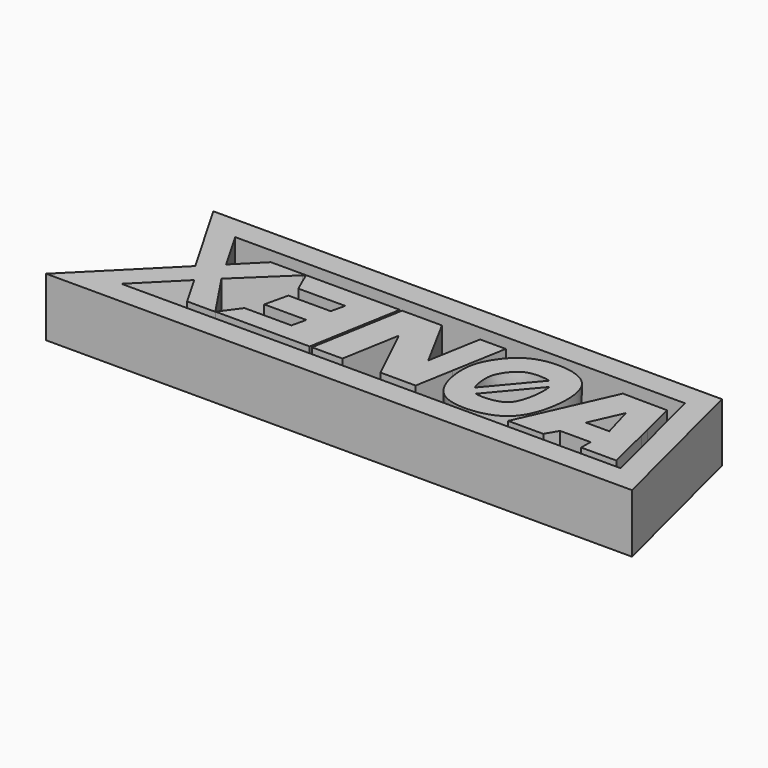
from build123d import *

# Parameters (mm, degrees)
F1_DEPTH = 25
F0_W     = 3.4720152617
F0_H     = 3.9200305776
F2_DEPTH = 15


# Not quite as in the source:
# - ends of sketch curves that miss each other by under 0.0002 mm in the source are joined
# - the dataset's text gives a spline's control points without its knots; the knots are read off the source's solid
# - a feature names something its author has since deleted; it is built from what else it names


with BuildPart() as f1:
    # F0 (on Top) → F1 (new body)
    with BuildSketch(Plane.XY):
        Polygon((35.3553390593, 35.3553390593), (0, 0), (250, 0), (232.3553390593, 69.9963552107), (15.3553390593, 69.9963552107), align=None)
        Polygon((149.3519097567, 59.9963530121), (224.56330661, 59.9963530121), (230.3136809852, 37.1846226695), (231.3968486735, 32.8876973548), (237.166372237, 10.0000021986), (140.1480585337, 10.0000021986), (136.676043272, 10.0000021986), (24.1421409317, 10.0000021986), (41.4001874912, 27.2580487582), (47.8522307846, 33.7100920516), (42.6758487445, 42.6758487445), (32.6758509431, 59.9963530121), (146.3302671909, 59.9963530121), align=None, mode=Mode.SUBTRACT)
        Polygon((53.2824504623, 53.2824504623), (42.6758487445, 42.6758487445), (47.8522307846, 33.7100920516), (67.4404504829, 52.4758059113), (68.2824504623, 53.2824504623), align=None)
        Polygon((60.8468717116, 14.278005959), (47.8522307846, 33.7100920516), (41.4001874912, 27.2580487582), (49.1933937334, 13.7598195929), (61.1933937334, 13.7598195929), align=None)
    extrude(amount=F1_DEPTH)


with BuildPart() as f1b:
    # F0 (on Top) → F1, piece 2 (new body)
    with BuildSketch(Plane.XY):
        Polygon((88.5540837341, 28.1308456181), (90.9036234209, 38.1308456181), (72.9036234209, 38.1308456181), (70.5540837341, 28.1308456181), align=None)
        Polygon((108.2824504623, 53.2824504623), (68.2824504623, 53.2824504623), (68.6377434378, 52.4758059113), (72.313347233, 44.1308456181), (92.313347233, 44.1308456181), (90.9036234209, 38.1308456181), (88.5540837341, 28.1308456181), (87.1034676285, 21.9568017674), (67.1034676285, 21.9568017674), (61.477565132, 14.278005959), (61.1933937334, 13.8901403418), (101.3365233556, 13.8901403418), align=None)
    extrude(amount=F1_DEPTH)



with BuildPart() as f1c:
    # F0 (on Top) → F1, piece 3 (new body)
    with BuildSketch(Plane.XY):
        Polygon((153.4814404268, 53.3123428967), (149.3519097567, 53.3123428967), (146.5191096067, 53.3123428967), (142.5191015005, 53.3123428967), (138.5251934142, 30.6617645774), (126.2824504623, 53.2824504623), (109.2824504623, 53.2824504623), (102.3365233556, 13.8901403418), (115.3365233556, 13.8901403418), (119.6777277973, 38.5103341671), (131.5355133201, 13.9200327762), (136.676043272, 13.9200327762), (140.1480585337, 13.9200327762), (146.5355133201, 13.9200327762), (149.3944048747, 30.1336124743), (151.5543764817, 42.3834201799), align=None)
    extrude(amount=F1_DEPTH)


with BuildPart() as f1d:
    # F0 (on Top) → F1, piece 4 (new body)
    with BuildSketch(Plane.XY):
        with BuildLine():
            add(Edge.make_bspline(
                [(153.2957728652, 41.0807725054), (153.49766281, 41.5309282211), (155.3500865512, 45.3378659555), (161.5552143615, 53.4867465492), (176.1548241084, 56.3217499328), (193.5548048204, 51.0510310034), (192.6995287251, 33.1029715051), (190.5478645245, 26.016644206)],
                knots=[0.0743708641, 0.0743708641, 0.0743708641, 0.0743708641, 0.0883183193, 0.1917010674, 0.3023367007, 0.4162516271, 0.5490950731, 0.5490950731, 0.5490950731, 0.5490950731], degree=3))
            add(Edge.make_bspline(
                [(151.5315026045, 33.6161878365), (151.6634499925, 36.3480245715), (152.2192517782, 38.6804443414), (153.2957728652, 41.0807725054)],
                knots=[0, 0, 0, 0, 0.0743708641, 0.0743708641, 0.0743708641, 0.0743708641], degree=3))
            add(Edge.make_bspline(
                [(151.5581660211, 30.4933039686), (151.4916370849, 31.5702465606), (151.4833764702, 32.6197850769), (151.5315026045, 33.6161878365)],
                knots=[0.9728741717, 0.9728741717, 0.9728741717, 0.9728741717, 1, 1, 1, 1], degree=3))
            add(Edge.make_bspline(
                [(188.4193204432, 20.8541177869), (186.4225620314, 17.2582664486), (179.6863041093, 11.4034157724), (160.3055787763, 10.4275817806), (153.2214749313, 20.0421386094), (151.7433054324, 27.4963446143), (151.5581660211, 30.4933039686)],
                knots=[0.5854070027, 0.5854070027, 0.5854070027, 0.5854070027, 0.6722296295, 0.7975352428, 0.8973873208, 0.9728741717, 0.9728741717, 0.9728741717, 0.9728741717], degree=3))
            add(Edge.make_bspline(
                [(190.5478645245, 26.016644206), (190.3967980643, 25.5191193687), (189.7761974015, 23.6315541865), (189.0399275657, 21.9717346898), (188.4193204432, 20.8541177869)],
                knots=[0.5490950731, 0.5490950731, 0.5490950731, 0.5490950731, 0.5584218951, 0.5854070027, 0.5854070027, 0.5854070027, 0.5854070027], degree=3))
        make_face()
        with BuildLine():
            add(Edge.make_bspline(
                [(162.8184250503, 25.0692523461), (162.7388528349, 25.2709199434), (162.5250729743, 25.8491123795), (162.2111113791, 26.8772771924), (161.811446171, 28.5859325459), (161.5680124914, 30.3698864013), (161.490617043, 32.0313577817), (161.5032118997, 32.7877081125), (161.5198585813, 33.1337514359)],
                knots=[0.8971962129, 0.8971962129, 0.8971962129, 0.8971962129, 0.90625, 0.921875, 0.9375, 0.96875, 0.984375, 1, 1, 1, 1], degree=3))
            add(Edge.make_bspline(
                [(161.5198585813, 33.1337514359), (161.5365052629, 33.4797947593), (161.5904971328, 34.1076177221), (161.7198338174, 34.8971109654), (161.8983772283, 35.617959176), (162.1037900469, 36.2305480911), (162.3191108206, 36.7643620724), (162.5109148317, 37.1933987719), (162.7379267984, 37.6574642255), (163.0921353714, 38.326605495), (163.596210236, 39.1811127594), (164.287470415, 40.1970519056), (165.0414513207, 41.1551577869), (165.8327231283, 42.017135319), (166.4983498938, 42.6285934344), (167.0176778213, 43.0428000772), (167.3981141086, 43.3156806379), (167.7595288983, 43.5467960735), (168.1488651256, 43.766963423), (168.5654607343, 43.9738592368), (169.1603655772, 44.23185257), (169.9804869671, 44.5178805652), (171.0896341478, 44.7915612101), (172.3184150489, 44.9834054828), (173.6559028444, 45.0826399089), (174.7295299917, 45.0813201083), (175.4692709806, 45.0471315589), (175.9685909899, 45.0153875781), (176.5764482855, 44.960404607), (177.2752413398, 44.8700053931), (178.152789541, 44.7188709988), (178.7412145092, 44.5732668808), (179.0910574906, 44.4674492213), (179.0945257888, 44.4663980322)],
                knots=[0, 0, 0, 0, 0.015625, 0.03125, 0.046875, 0.0625, 0.0703125, 0.078125, 0.0859375, 0.09375, 0.109375, 0.125, 0.140625, 0.15625, 0.171875, 0.1796875, 0.1875, 0.1953125, 0.203125, 0.2109375, 0.21875, 0.234375, 0.25, 0.265625, 0.28125, 0.296875, 0.30078125, 0.3046875, 0.3125, 0.3203125, 0.328125, 0.34375, 0.3439066519, 0.3439066519, 0.3439066519, 0.3439066519], degree=3))
            add(Edge.make_bspline(
                [(179.0945257888, 44.4663980322), (179.4369974189, 44.3626000224), (180.0408289592, 44.137858269), (180.6603332198, 43.8043498556), (180.954614815, 43.5775919437), (181.1038370269, 43.4315691806), (181.1895827034, 43.3310307887), (181.2538264485, 43.2395291398), (181.3046724038, 43.1550069204), (181.3582155541, 43.05569095), (181.422796919, 42.9212624239), (181.5199173994, 42.6948431225), (181.7085595453, 42.1772024114), (181.8753089955, 41.5231873988), (181.9696544415, 41.0096622148), (181.9730783847, 40.9907957298)],
                knots=[0.3439066519, 0.3439066519, 0.3439066519, 0.3439066519, 0.359375, 0.375, 0.390625, 0.3984375, 0.40625, 0.4140625, 0.41796875, 0.421875, 0.42578125, 0.4296875, 0.4375, 0.453125, 0.4537178211, 0.4537178211, 0.4537178211, 0.4537178211], degree=3))
            add(Edge.make_bspline(
                [(181.9730783847, 40.9907957298), (182.0598994005, 40.512397778), (182.2045363428, 39.41183358), (182.2797979507, 37.4823107399), (182.193566141, 35.3678582229), (181.9493626032, 33.2017921364), (181.5644163989, 31.0887847577), (181.0667847965, 29.1323622869), (180.5011449009, 27.4494312491), (179.9317447836, 26.1476864655), (179.3824865747, 25.1785905134), (178.8685398921, 24.4779841747), (178.3709172748, 23.9520794031), (177.8264944089, 23.5060953751), (177.1374617731, 23.0738355235), (176.2112022482, 22.6358864412), (174.9558716393, 22.2007569681), (173.4559950281, 21.8323747048), (171.8198374216, 21.5722282716), (170.1442177268, 21.4412866926), (168.5280439261, 21.4466193999), (167.3160139795, 21.558065936), (166.4822451641, 21.6958640201), (166.0986472535, 21.7808626756), (165.9163137021, 21.8272428827), (165.8971010414, 21.8322026836)],
                knots=[0.4537178211, 0.4537178211, 0.4537178211, 0.4537178211, 0.46875, 0.484375, 0.5, 0.515625, 0.53125, 0.546875, 0.5625, 0.578125, 0.59375, 0.609375, 0.625, 0.640625, 0.65625, 0.671875, 0.6875, 0.703125, 0.71875, 0.734375, 0.75, 0.765625, 0.7734375, 0.78125, 0.7821827292, 0.7821827292, 0.7821827292, 0.7821827292], degree=3))
            add(Edge.make_bspline(
                [(165.8971010414, 21.8322026836), (165.7553892759, 21.868785963), (165.5531970067, 21.9272567748), (165.3254056153, 22.0041417656), (165.1739060305, 22.0612615773), (165.0494707627, 22.1134592968), (164.8977695401, 22.1837784003), (164.7376634219, 22.2699020236), (164.5740601511, 22.3743238889), (164.3757102389, 22.5229923761), (164.1329229874, 22.7478764528), (163.795317607, 23.1578632169), (163.4078371213, 23.7696356085), (163.0732924198, 24.4470716455), (162.8761783378, 24.9228825776), (162.8184250503, 25.0692523461)],
                knots=[0.7821827292, 0.7821827292, 0.7821827292, 0.7821827292, 0.7890625, 0.79296875, 0.796875, 0.80078125, 0.8046875, 0.8125, 0.8203125, 0.828125, 0.84375, 0.859375, 0.875, 0.890625, 0.8971962129, 0.8971962129, 0.8971962129, 0.8971962129], degree=3))
        make_face(mode=Mode.SUBTRACT)
        with BuildLine():
            add(Edge.make_bspline(
                [(179.0945257888, 44.4663980322), (179.4369974189, 44.3626000224), (180.0408289592, 44.137858269), (180.6603332198, 43.8043498556), (180.954614815, 43.5775919437), (181.1038370269, 43.4315691806), (181.1895827034, 43.3310307887), (181.2538264485, 43.2395291398), (181.3046724038, 43.1550069204), (181.3582155541, 43.05569095), (181.422796919, 42.9212624239), (181.5199173994, 42.6948431225), (181.7085595453, 42.1772024114), (181.8753089955, 41.5231873988), (181.9696544415, 41.0096622148), (181.9730783847, 40.9907957298)],
                knots=[0.3439066519, 0.3439066519, 0.3439066519, 0.3439066519, 0.359375, 0.375, 0.390625, 0.3984375, 0.40625, 0.4140625, 0.41796875, 0.421875, 0.42578125, 0.4296875, 0.4375, 0.453125, 0.4537178211, 0.4537178211, 0.4537178211, 0.4537178211], degree=3))
            Line((179.0945257888, 44.4663980322), (162.8183697977, 25.0692305451))
            add(Edge.make_bspline(
                [(165.8971010414, 21.8322026836), (165.7553892759, 21.868785963), (165.5531970067, 21.9272567748), (165.3254056153, 22.0041417656), (165.1739060305, 22.0612615773), (165.0494707627, 22.1134592968), (164.8977695401, 22.1837784003), (164.7376634219, 22.2699020236), (164.5740601511, 22.3743238889), (164.3757102389, 22.5229923761), (164.1329229874, 22.7478764528), (163.795317607, 23.1578632169), (163.4078371213, 23.7696356085), (163.0732924198, 24.4470716455), (162.8761783378, 24.9228825776), (162.8183697977, 25.0692305451)],
                knots=[0.7821827292, 0.7821827292, 0.7821827292, 0.7821827292, 0.7890625, 0.79296875, 0.796875, 0.80078125, 0.8046875, 0.8125, 0.8203125, 0.828125, 0.84375, 0.859375, 0.875, 0.890625, 0.8971962129, 0.8971962129, 0.8971962129, 0.8971962129], degree=3))
            Line((165.8971010414, 21.8322026836), (181.9730783847, 40.9907957298))
        make_face()
    extrude(amount=F1_DEPTH)


with BuildPart() as f1e:
    # F0 (on Top) → F1, piece 5 (new body)
    with BuildSketch(Plane.XY):
        Polygon((227.8092346476, 32.8876973548), (226.7642129222, 37.1846226695), (223.0829559751, 52.321232543), (204.0839364723, 52.5142556785), (192.2389093289, 26.016644206), (189.1953905746, 19.20821933), (186.5355133201, 13.258009744), (201.5355133201, 13.258009744), (204.5355133201, 18.4541621667), (217.5355133201, 18.4541621667), (217.5355133201, 13.4541621667), (232.5355133201, 13.4541621667), align=None)
        Polygon((213.6570562804, 42.148201446), (217.5355133201, 28.4541621667), (207.5355133201, 28.4541621667), align=None, mode=Mode.SUBTRACT)
    extrude(amount=F1_DEPTH)


with BuildPart() as f1b_1:
    add(f1b.part)

    add(f1c.part)  # F2 merges F1c

    add(f1d.part)  # F2 merges F1d

    add(f1e.part)  # F2 merges F1e
    # F0 (on Top) → F2 (join)
    with BuildSketch(Plane.XY):
        Polygon((149.3519097567, 53.3123428967), (149.3519097567, 59.9963530121), (146.3302671909, 59.9963530121), (146.5191096067, 53.3123428967), align=None)
        with Locations((138.4120509028, 11.9600174874)):
            Rectangle(F0_W, F0_H)
        with BuildLine():
            Line((153.2957728652, 41.0807725054), (151.5543764817, 42.3834201799))
            Line((151.5543764817, 42.3834201799), (149.3944048747, 30.1336124743))
            Line((149.3944048747, 30.1336124743), (151.5581660211, 30.4933039686))
            add(Edge.make_bspline(
                [(151.5581660211, 30.4933039686), (151.4916370849, 31.5702465606), (151.4833764702, 32.6197850769), (151.5315026045, 33.6161878365)],
                knots=[0.9728741717, 0.9728741717, 0.9728741717, 0.9728741717, 1, 1, 1, 1], degree=3))
            add(Edge.make_bspline(
                [(151.5315026045, 33.6161878365), (151.6634499925, 36.3480245715), (152.2192517782, 38.6804443414), (153.2957728652, 41.0807725054)],
                knots=[0, 0, 0, 0, 0.0743708641, 0.0743708641, 0.0743708641, 0.0743708641], degree=3))
        make_face()
        with BuildLine():
            Line((189.1953905746, 19.20821933), (192.2389093289, 26.016644206))
            Line((192.2389093289, 26.016644206), (190.5478645245, 26.016644206))
            add(Edge.make_bspline(
                [(190.5478645245, 26.016644206), (190.3967980643, 25.5191193687), (189.7761974015, 23.6315541865), (189.0399275657, 21.9717346898), (188.4193204432, 20.8541177869)],
                knots=[0.5490950731, 0.5490950731, 0.5490950731, 0.5490950731, 0.5584218951, 0.5854070027, 0.5854070027, 0.5854070027, 0.5854070027], degree=3))
            Line((188.4193204432, 20.8541177869), (189.1953905746, 19.20821933))
        make_face()
        Polygon((231.3968486735, 32.8876973548), (230.3136809852, 37.1846226695), (226.7642129222, 37.1846226695), (227.8092346476, 32.8876973548), align=None)
        Polygon((109.2824504623, 53.2824504623), (108.2824504623, 53.2824504623), (101.3365233556, 13.8901403418), (102.3365233556, 13.8901403418), align=None)
        Polygon((61.477565132, 14.278005959), (60.8468717116, 14.278005959), (61.1933937334, 13.7598195929), (61.1933937334, 13.8901403418), align=None)
        Polygon((68.2824504623, 53.2824504623), (67.4404504829, 52.4758059113), (68.6377434378, 52.4758059113), align=None)
    extrude(amount=F2_DEPTH)


solid = Compound([f1.part, f1b_1.part])
